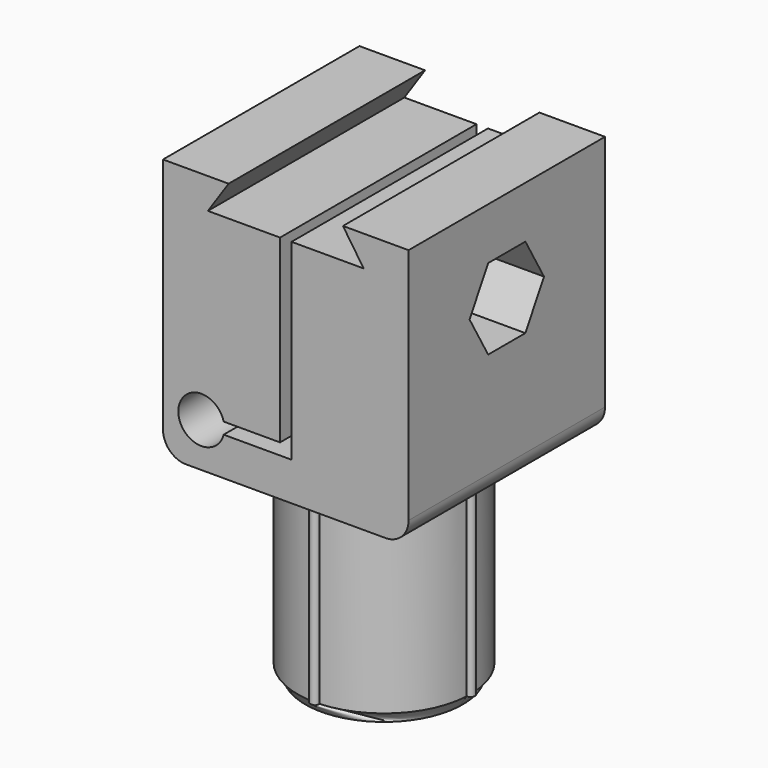
from build123d import *

# Parameters (mm, degrees)
F1_DEPTH  = 32
F2_R      = 6
F3_DEPTH  = 10
F4_R      = 3.4
F5_DEPTH  = 22.001
F7_DEPTH  = 32.001
F9_DEPTH  = 11
F11_DEPTH = 25
F12_R     = 3
F13_R     = 3


# Not quite as in the source:
# - the arcs of a loft's sections are written as splines that run evenly, so that the points pair up as in the source's solid


with BuildPart() as f1:
    # F0 (on Front) → F1 (new body)
    with BuildSketch(Plane.XZ):
        Polygon((-16, 17), (-16, -17), (16, -17), (16, 17), (7.4519659326, 17), (10.15, 13), (-10.15, 13), (-7.4519659326, 17), align=None)
    extrude(amount=F1_DEPTH)

    # F2 (on face) → F3 (cut)
    with BuildSketch(Plane(origin=(-16, 0, 0), x_dir=(0, -1, 0), z_dir=(-1, 0, 0))):
        with Locations((16, 5)):
            Circle(F2_R)
    extrude(amount=-F3_DEPTH, mode=Mode.SUBTRACT)

    # F4 (on face) → F5 (cut, through all)
    with BuildSketch(Plane(origin=(-6, 0, 0), x_dir=(0, -1, 0), z_dir=(-1, 0, 0))):
        with Locations((16, 5)):
            Circle(F4_R)
    extrude(amount=-F5_DEPTH, mode=Mode.SUBTRACT)

    # F6 (on face) → F7 (cut, through all)
    with BuildSketch(Plane.XZ.offset(32)):
        with BuildLine():
            Line((0.75, 13), (-0.75, 13))
            Line((-0.75, 13), (-0.75, -10.5))
            Line((-0.75, -10.5), (-8.0952624903, -10.5))
            ThreePointArc((-8.0952624903, -10.5), (-14, -11.25), (-8.0952624903, -12))
            Line((-8.0952624903, -12), (0.75, -12))
            Line((0.75, -12), (0.75, 13))
        make_face()
    extrude(amount=-F7_DEPTH, mode=Mode.SUBTRACT)

    # F8 (on face) → F9 (cut)
    with BuildSketch(Plane.YZ.offset(16)):
        Polygon((-12.9689110868, -0.25), (-9.9378221735, 5), (-12.9689110868, 10.25), (-19.0310889132, 10.25), (-22.0621778265, 5), (-19.0310889132, -0.25), align=None)
    extrude(amount=-F9_DEPTH, mode=Mode.SUBTRACT)

    # F10 (on face) → F11 (join)
    with BuildSketch(Plane(origin=(0, 0, -17), x_dir=(1, 0, 0), z_dir=(0, 0, -1))):
        with BuildLine():
            ThreePointArc((11.234, 15.4002133713), (11.85, 16), (11.234, 16.5997866287))
            ThreePointArc((11.234, 16.5997866287), (7.9549512883, 23.9549512883), (0.5997866287, 27.234))
            ThreePointArc((0.5997866287, 27.234), (0, 27.85), (-0.5997866287, 27.234))
            ThreePointArc((-0.5997866287, 27.234), (-7.9549512883, 23.9549512883), (-11.234, 16.5997866287))
            ThreePointArc((-11.234, 16.5997866287), (-11.85, 16), (-11.234, 15.4002133713))
            ThreePointArc((-11.234, 15.4002133713), (-7.9549512883, 8.0450487117), (-0.5997866287, 4.766))
            ThreePointArc((-0.5997866287, 4.766), (0, 4.15), (0.5997866287, 4.766))
            ThreePointArc((0.5997866287, 4.766), (7.9549512883, 8.0450487117), (11.234, 15.4002133713))
        make_face()
    extrude(amount=F11_DEPTH)

    # F12
    f12_edges = [f1.edges().sort_by_distance(p)[0] for p in [
        (-16, -16, -17),
    ]]
    fillet(f12_edges, radius=F12_R)

    # F13
    f13_edges = [f1.edges().sort_by_distance(p)[0] for p in [
        (16, -16, -17),
    ]]
    fillet(f13_edges, radius=F13_R)

    # F11_face (on face) → F16 section 0
    with BuildSketch(Plane(origin=(0, -16, -42), x_dir=(1, 0, 0), z_dir=(0, 0, -1))):
        with BuildLine():
            add(Edge.make_bspline(
                [(0.5997866287, -11.234), (1.9704441734, -11.1608201827), (3.3271537618, -10.8340484232), (5.834489174, -9.7162386482), (6.984369661, -8.9255329157), (8.9255329157, -6.984369661), (9.7162386482, -5.834489174), (10.8340484232, -3.3271537618), (11.1608201827, -1.9704441734), (11.234, -0.5997866287)],
                knots=[0, 0, 0, 0, 0.25, 0.25, 0.5, 0.5, 0.75, 0.75, 1, 1, 1, 1], degree=3))
            add(Edge.make_bspline(
                [(11.234, -0.5997866287), (11.3049732474, -0.6016799219), (11.376267359, -0.5908445992), (11.5106795168, -0.5450568557), (11.5737621993, -0.5101164815), (11.6838785828, -0.4204642218), (11.7308833124, -0.3657759235), (11.8029722112, -0.2434389451), (11.8280374139, -0.1758224517), (11.853109213, -0.0360563953), (11.853109213, 0.0360563953), (11.8280374139, 0.1758224517), (11.8029722112, 0.2434389451), (11.7308833124, 0.3657759235), (11.6838785828, 0.4204642218), (11.5737621993, 0.5101164815), (11.5106795168, 0.5450568557), (11.376267359, 0.5908445992), (11.3049732474, 0.6016799219), (11.234, 0.5997866287)],
                knots=[0, 0, 0, 0, 0.1111111111, 0.1111111111, 0.2222222222, 0.2222222222, 0.3333333333, 0.3333333333, 0.4444444444, 0.4444444444, 0.5555555556, 0.5555555556, 0.6666666667, 0.6666666667, 0.7777777778, 0.7777777778, 0.8888888889, 0.8888888889, 1, 1, 1, 1], degree=3))
            add(Edge.make_bspline(
                [(11.234, 0.5997866287), (11.1608201827, 1.9704441734), (10.8340484232, 3.3271537618), (9.7162386482, 5.834489174), (8.9255329157, 6.984369661), (6.984369661, 8.9255329157), (5.834489174, 9.7162386482), (3.3271537618, 10.8340484232), (1.9704441734, 11.1608201827), (0.5997866287, 11.234)],
                knots=[0, 0, 0, 0, 0.25, 0.25, 0.5, 0.5, 0.75, 0.75, 1, 1, 1, 1], degree=3))
            add(Edge.make_bspline(
                [(0.5997866287, 11.234), (0.6016799219, 11.3049732474), (0.5908445992, 11.376267359), (0.5450568557, 11.5106795168), (0.5101164815, 11.5737621993), (0.4204642218, 11.6838785828), (0.3657759235, 11.7308833124), (0.2434389451, 11.8029722112), (0.1758224517, 11.8280374139), (0.0360563953, 11.853109213), (-0.0360563953, 11.853109213), (-0.1758224517, 11.8280374139), (-0.2434389451, 11.8029722112), (-0.3657759235, 11.7308833124), (-0.4204642218, 11.6838785828), (-0.5101164815, 11.5737621993), (-0.5450568557, 11.5106795168), (-0.5908445992, 11.376267359), (-0.6016799219, 11.3049732474), (-0.5997866287, 11.234)],
                knots=[0, 0, 0, 0, 0.1111111111, 0.1111111111, 0.2222222222, 0.2222222222, 0.3333333333, 0.3333333333, 0.4444444444, 0.4444444444, 0.5555555556, 0.5555555556, 0.6666666667, 0.6666666667, 0.7777777778, 0.7777777778, 0.8888888889, 0.8888888889, 1, 1, 1, 1], degree=3))
            add(Edge.make_bspline(
                [(-0.5997866287, 11.234), (-1.9704441734, 11.1608201827), (-3.3271537618, 10.8340484232), (-5.834489174, 9.7162386482), (-6.984369661, 8.9255329157), (-8.9255329157, 6.984369661), (-9.7162386482, 5.834489174), (-10.8340484232, 3.3271537618), (-11.1608201827, 1.9704441734), (-11.234, 0.5997866287)],
                knots=[0, 0, 0, 0, 0.25, 0.25, 0.5, 0.5, 0.75, 0.75, 1, 1, 1, 1], degree=3))
            add(Edge.make_bspline(
                [(-11.234, 0.5997866287), (-11.3049732474, 0.6016799219), (-11.376267359, 0.5908445992), (-11.5106795168, 0.5450568557), (-11.5737621993, 0.5101164815), (-11.6838785828, 0.4204642218), (-11.7308833124, 0.3657759235), (-11.8029722112, 0.2434389451), (-11.8280374139, 0.1758224517), (-11.853109213, 0.0360563953), (-11.853109213, -0.0360563953), (-11.8280374139, -0.1758224517), (-11.8029722112, -0.2434389451), (-11.7308833124, -0.3657759235), (-11.6838785828, -0.4204642218), (-11.5737621993, -0.5101164815), (-11.5106795168, -0.5450568557), (-11.376267359, -0.5908445992), (-11.3049732474, -0.6016799219), (-11.234, -0.5997866287)],
                knots=[0, 0, 0, 0, 0.1111111111, 0.1111111111, 0.2222222222, 0.2222222222, 0.3333333333, 0.3333333333, 0.4444444444, 0.4444444444, 0.5555555556, 0.5555555556, 0.6666666667, 0.6666666667, 0.7777777778, 0.7777777778, 0.8888888889, 0.8888888889, 1, 1, 1, 1], degree=3))
            add(Edge.make_bspline(
                [(-11.234, -0.5997866287), (-11.1608201827, -1.9704441734), (-10.8340484232, -3.3271537618), (-9.7162386482, -5.834489174), (-8.9255329157, -6.984369661), (-6.984369661, -8.9255329157), (-5.834489174, -9.7162386482), (-3.3271537618, -10.8340484232), (-1.9704441734, -11.1608201827), (-0.5997866287, -11.234)],
                knots=[0, 0, 0, 0, 0.25, 0.25, 0.5, 0.5, 0.75, 0.75, 1, 1, 1, 1], degree=3))
            add(Edge.make_bspline(
                [(-0.5997866287, -11.234), (-0.6016799219, -11.3049732474), (-0.5908445992, -11.376267359), (-0.5450568557, -11.5106795168), (-0.5101164815, -11.5737621993), (-0.4204642218, -11.6838785828), (-0.3657759235, -11.7308833124), (-0.2434389451, -11.8029722112), (-0.1758224517, -11.8280374139), (-0.0360563953, -11.853109213), (0.0360563953, -11.853109213), (0.1758224517, -11.8280374139), (0.2434389451, -11.8029722112), (0.3657759235, -11.7308833124), (0.4204642218, -11.6838785828), (0.5101164815, -11.5737621993), (0.5450568557, -11.5106795168), (0.5908445992, -11.376267359), (0.6016799219, -11.3049732474), (0.5997866287, -11.234)],
                knots=[0, 0, 0, 0, 0.1111111111, 0.1111111111, 0.2222222222, 0.2222222222, 0.3333333333, 0.3333333333, 0.4444444444, 0.4444444444, 0.5555555556, 0.5555555556, 0.6666666667, 0.6666666667, 0.7777777778, 0.7777777778, 0.8888888889, 0.8888888889, 1, 1, 1, 1], degree=3))
        make_face()
    # F15 (on offset) → F16 section 1
    with BuildSketch(Plane(origin=(0, 0, -43.5), x_dir=(1, 0, 0), z_dir=(0, 0, -1))):
        with BuildLine():
            add(Edge.make_bspline(
                [(0.5464722617, 5.7645777778), (1.8862858976, 5.8361108296), (3.2113491637, 6.1740163798), (5.6322529271, 7.3316411864), (6.7271409022, 8.1509049669), (7.6239507036, 9.1488777804)],
                knots=[0, 0, 0, 0, 0.5, 0.5, 1, 1, 1, 1], degree=3))
            add(Edge.make_bspline(
                [(7.6239507036, 9.1488777804), (8.5207605051, 10.1468505938), (9.2187864201, 11.3227471207), (10.112059537, 13.8531489393), (10.306955274, 15.2066586259), (10.2354222222, 16.5464722617)],
                knots=[0, 0, 0, 0, 0.5, 0.5, 1, 1, 1, 1], degree=3))
            add(Edge.make_bspline(
                [(10.2354222222, 16.5464722617), (10.1638891704, 17.8862858976), (9.8259836202, 19.2113491637), (8.6683588136, 21.6322529271), (7.8490950331, 22.7271409022), (6.8511222196, 23.6239507036)],
                knots=[0, 0, 0, 0, 0.5, 0.5, 1, 1, 1, 1], degree=3))
            add(Edge.make_bspline(
                [(6.8511222196, 23.6239507036), (5.8531494062, 24.5207605051), (4.6772528793, 25.2187864201), (2.1468510607, 26.112059537), (0.7933413741, 26.306955274), (-0.5464722617, 26.2354222222)],
                knots=[0, 0, 0, 0, 0.5, 0.5, 1, 1, 1, 1], degree=3))
            add(Edge.make_bspline(
                [(-0.5464722617, 26.2354222222), (-1.8862858976, 26.1638891704), (-3.2113491637, 25.8259836202), (-5.6322529271, 24.6683588136), (-6.7271409022, 23.8490950331), (-7.6239507036, 22.8511222196)],
                knots=[0, 0, 0, 0, 0.5, 0.5, 1, 1, 1, 1], degree=3))
            add(Edge.make_bspline(
                [(-7.6239507036, 22.8511222196), (-8.5207605051, 21.8531494062), (-9.2187864201, 20.6772528793), (-10.112059537, 18.1468510607), (-10.306955274, 16.7933413741), (-10.2354222222, 15.4535277383)],
                knots=[0, 0, 0, 0, 0.5, 0.5, 1, 1, 1, 1], degree=3))
            add(Edge.make_bspline(
                [(-10.2354222222, 15.4535277383), (-10.1638891704, 14.1137141024), (-9.8259836202, 12.7886508363), (-8.6683588136, 10.3677470729), (-7.8490950331, 9.2728590978), (-6.8511222196, 8.3760492964)],
                knots=[0, 0, 0, 0, 0.5, 0.5, 1, 1, 1, 1], degree=3))
            add(Edge.make_bspline(
                [(-6.8511222196, 8.3760492964), (-5.8531494062, 7.4792394949), (-4.6772528793, 6.7812135799), (-2.1468510607, 5.887940463), (-0.7933413741, 5.693044726), (0.5464722617, 5.7645777778)],
                knots=[0, 0, 0, 0, 0.5, 0.5, 1, 1, 1, 1], degree=3))
        make_face()
    loft(ruled=True)


solid = f1.part
